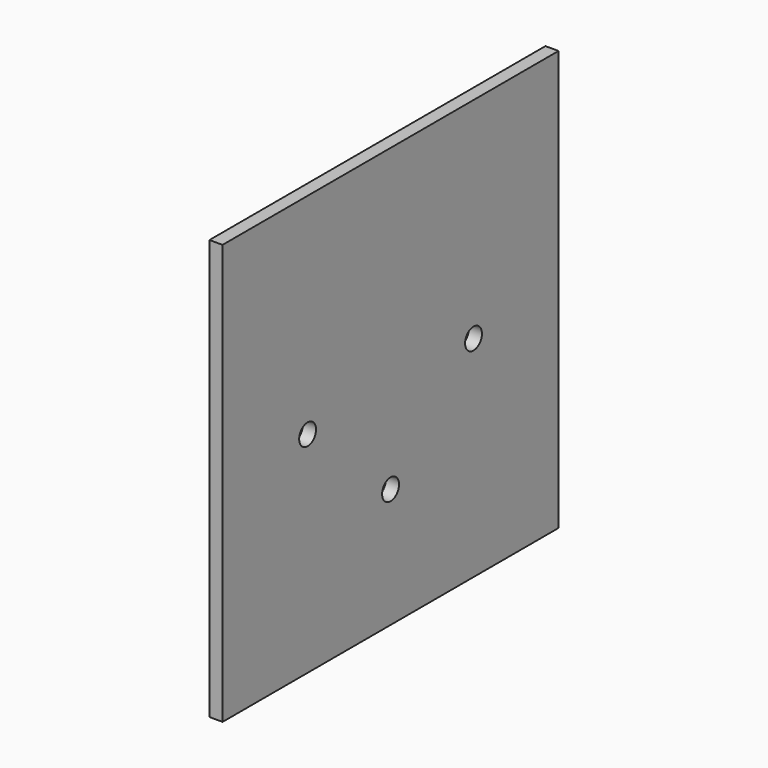
from build123d import *

# Parameters (mm, degrees)
F0_W     = 101.6
F0_H     = 101.6
F1_DEPTH = 3.175
F3_D     = 5.1054
F3_DEPTH = 25
F3_TIP   = 1.5338169022


# Not quite as in the source:
# - a length typed as a fraction of an inch, garbled in the dataset ("3 / 203.2 mm" for 3/8 in), is restored


with BuildPart() as f1:
    # F0 (on Right) → F1 (new body)
    with BuildSketch(Plane.YZ):
        Rectangle(F0_W, F0_H)
    extrude(amount=F1_DEPTH)

    # F3
    with Locations(Plane.YZ.offset(3.175)):
        with Locations((0, -21.9075), (-25.0825, 0), (25.0825, 0)):
            Hole(F3_D / 2, depth=F3_DEPTH)
            with Locations((0, 0, -(F3_DEPTH + F3_TIP / 2))):  # 118° drill point
                Cone(0, F3_D / 2, F3_TIP, mode=Mode.SUBTRACT)


solid = f1.part
